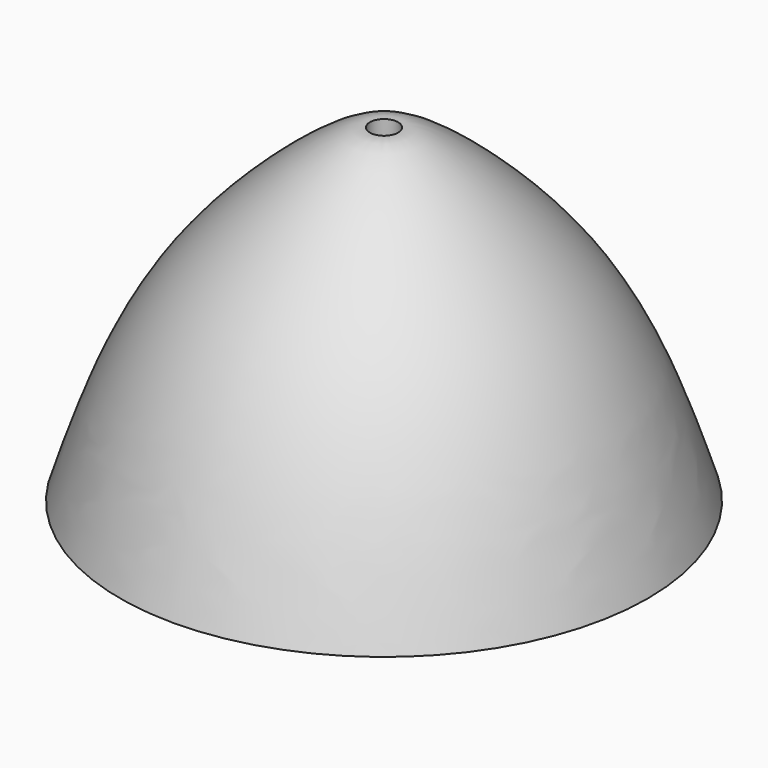
from build123d import *


# Not quite as in the source:
# - the dataset's text gives a spline's control points without its knots; the knots are read off the source's solid


with BuildPart() as f1:
    # F0 (on Right) → F1 (revolve)
    with BuildSketch(Plane.YZ):
        with BuildLine():
            add(Edge.make_bspline(
                [(-53.9826527238, 0), (-49.386958883, 14.2353536881), (-40.6217945453, 41.385816448), (-8.3411574095, 67.5468728143), (-3.9808685597, 67.2991772174), (-2.891927259, 67.2373175621)],
                knots=[0, 0, 0, 0, 0.4526409905, 0.8633022141, 1, 1, 1, 1], degree=3))
            Line((-53.9826527238, 0), (-47.9397551579, -1.9508687829))
            add(Edge.make_bspline(
                [(-47.9397551579, -1.9508687829), (-46.6706219108, 1.9803244766), (-44.7925139615, 7.7934810315), (-42.0212182178, 15.3055097556), (-39.7340017165, 20.8063102799), (-37.1632728164, 26.1636626482), (-34.722102345, 30.504430212), (-32.5501607968, 33.9028221407), (-30.8016833685, 36.4150792356), (-28.9210935447, 38.890585225), (-26.8889002003, 41.3561448458), (-24.7461569978, 43.7782808482), (-21.7837472678, 46.9197566327), (-17.9685538725, 50.6212158674), (-14.2307427496, 53.8713931373), (-11.431229937, 56.1098430679), (-9.4667524013, 57.5838227792), (-7.6819625754, 58.8272714486), (-6.389339767, 59.6473712834), (-5.5113861941, 60.1564234952), (-4.9457253468, 60.4596305484), (-4.4930858224, 60.6784735453), (-4.1822378998, 60.8087596755), (-3.9751059498, 60.8810153424), (-3.8651785566, 60.9106164831), (-3.8270674235, 60.9176546254), (-3.82519652, 60.9171423754), (-3.7981648641, 60.9237284548), (-3.5010111061, 60.9116802417), (-3.2520720939, 60.8975387254)],
                knots=[-1e-10, -1e-10, -1e-10, -1e-10, 0.1250000001, 0.1875000003, 0.2500000004, 0.3125000005, 0.3750000007, 0.4062500007, 0.4375000008, 0.4687500009, 0.5000000009, 0.531250001, 0.562500001, 0.6250000012, 0.6875000013, 0.7187500014, 0.7500000014, 0.7812500015, 0.8125000016, 0.8281250016, 0.8437500016, 0.8593750017, 0.8750000017, 0.8906250017, 0.9062500018, 0.9218750018, 0.9375000018, 0.9687500019, 1, 1, 1, 1], degree=3))
            Line((-3.252072047, 60.8975387228), (-2.891927259, 67.2373175621))
        make_face()
    revolve(axis=Axis((0, 0, 36.6310849786), (0, 0, 1)))


solid = f1.part
